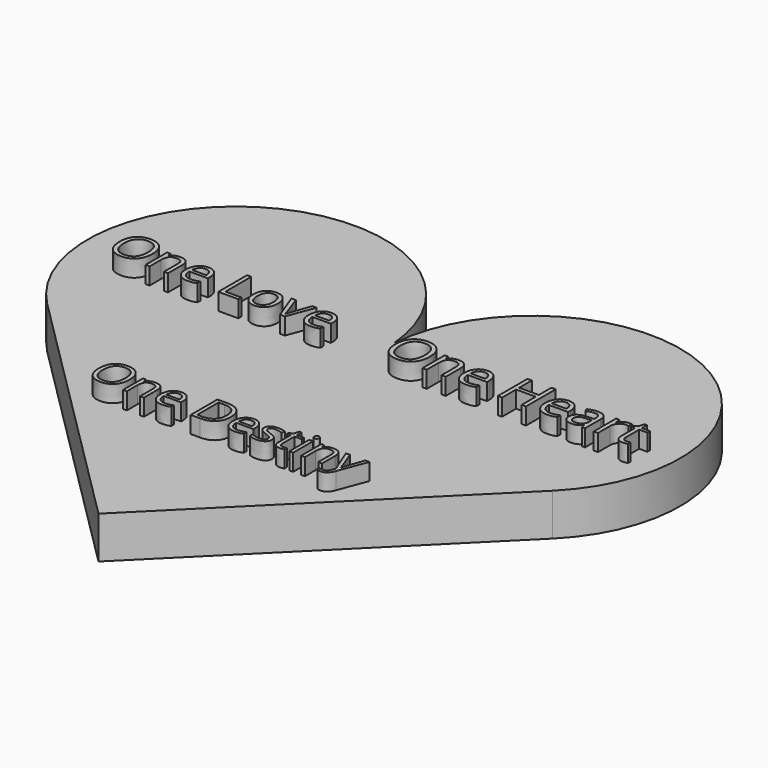
from build123d import *

# Parameters (mm, degrees)
F4_DEPTH     = 12.7
F1_TEXT_SIZE = 14.0897425202
F2_TEXT_SIZE = 15.1531175814
F3_TEXT_SIZE = 15.6848057587
F5_DEPTH     = 17.78


# Not quite as in the source:
# - Text() gives the source's letters only with a copy of the font that has no kerning and outlines rounded to 1/6400 em; it was checked with that copy


with BuildPart() as f4:
    # F0 (on Top) → F4 (new body)
    with BuildSketch(Plane.XY):
        with BuildLine():
            Line((-76.1006674644, 0), (0, -75.8450510941))
            Line((0, -75.8450510941), (76.104275655, 0))
            ThreePointArc((76.104275655, 0), (63.4571283378, 72.1817859257), (-0.0002297457, 35.5303976881))
            ThreePointArc((-0.0002297457, 35.5303976881), (-63.4543586567, 72.1763172241), (-76.1006674644, 0))
        make_face()
        with BuildLine():
            ThreePointArc((0, 27.8048831969), (-0.1672887009, 31.667635471), (-0.0002297457, 35.5303976881))
            ThreePointArc((-0.0002297457, 35.5303976881), (0.1670690289, 31.6676454143), (0, 27.8048831969))
        make_face(mode=Mode.SUBTRACT)
        with BuildLine():
            ThreePointArc((0, 27.8048831969), (0.1670690289, 31.6676454143), (-0.0002297457, 35.5303976881))
            ThreePointArc((-0.0002297457, 35.5303976881), (-0.1672887009, 31.667635471), (0, 27.8048831969))
        make_face()
    extrude(amount=F4_DEPTH)

    # F1 (on face) + F2 (on face) + F3 (on face) → F5 (join)
    with BuildSketch(Plane.XY):
        with Locations((-40.9586997703, -30.6312711909)):
            Text('One Destiny', F1_TEXT_SIZE, font='Open Sans', text_align=(TextAlign.LEFT, TextAlign.BOTTOM))
    with BuildSketch(Plane.XY):
        with Locations((-77.5175951421, 22.3886910826)):
            Text('One Love', F2_TEXT_SIZE, font='Open Sans', text_align=(TextAlign.LEFT, TextAlign.BOTTOM))
    with BuildSketch(Plane.XY):
        with Locations((5.7448036969, 22.0058755949)):
            Text('One Heart', F3_TEXT_SIZE, font='Open Sans', text_align=(TextAlign.LEFT, TextAlign.BOTTOM))
    extrude(amount=F5_DEPTH)


solid = f4.part
